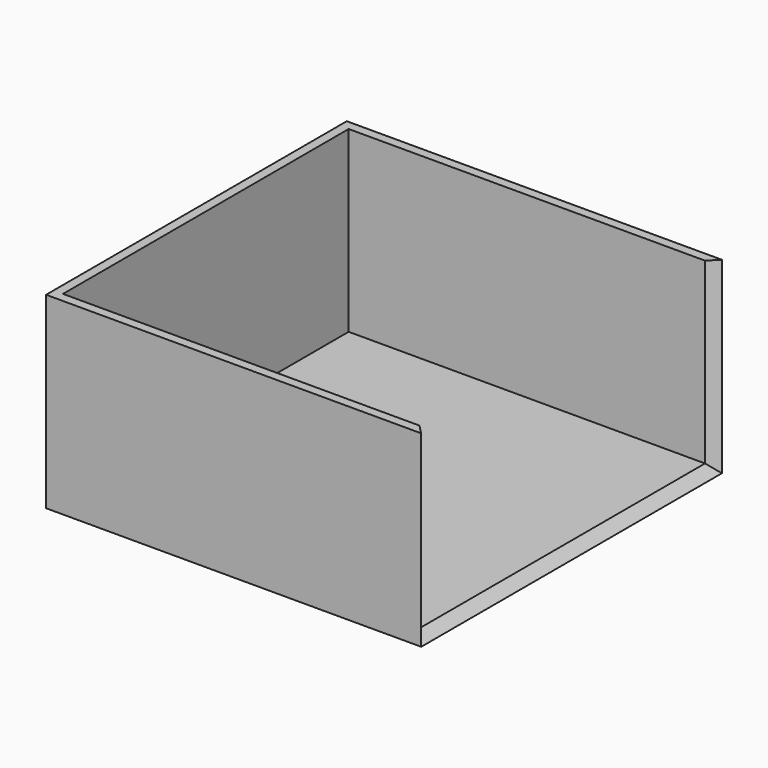
from build123d import *

# Parameters (mm, degrees)
F0_W         = 127
F0_H         = 127
F1_DEPTH     = 63.5
F2_W         = 120.65
F2_H         = 120.65
F2_W_2       = 40.16652188
F3_DEPTH     = 60.325
F4_T1_DEPTH  = 69.1433009657
F4_T3_DEPTH  = 120.65
F4_T9_DEPTH  = 129.4683009657
F4_T15_DEPTH = 69.1433009657
F4_T24_DEPTH = 69.1433009657
F4_T30_DEPTH = 129.4683009657


# Not quite as in the source:
# - a fillet or chamfer that OpenCascade refuses, or shapes differently, is made with other operations: its cross-section is extruded or revolved along the edge and cut away or added


with BuildPart() as f1:
    # F0 (on Top) → F1 (new body)
    with BuildSketch(Plane.XY):
        with Locations((9.8422262818, 3.4245376295)):
            Rectangle(F0_W, F0_H)
    extrude(amount=F1_DEPTH)

    # F2 (on face) → F3 (cut)
    with BuildSketch(Plane.XY.offset(63.5)):
        with Locations((9.8422262818, 3.4245376295)):
            Rectangle(F2_W, F2_H)
        with Locations((90.2504872218, 3.4245376295)):
            Rectangle(F2_W_2, F2_H)
    extrude(amount=-F3_DEPTH, mode=Mode.SUBTRACT)

    # F4: chamfer of 3.429 on 3 edges, made by hand

    # F4_s2 → F4_t1 (cut)
    with BuildSketch(Plane.XY.offset(3.175)):
        Polygon((73.3422262818, -60.3294623705), (69.9132262818, -56.9004623705), (73.3422262818, -56.9004623705), align=None)
        Polygon((73.3422262818, 67.1785376295), (69.9132262818, 63.7495376295), (73.3422262818, 63.7495376295), align=None)
    extrude(amount=F4_T1_DEPTH, mode=Mode.SUBTRACT)

    # F4_s4 → F4_t3 (cut)
    with BuildSketch(Plane.XZ.offset(-63.7495376295)):
        Polygon((73.3422262818, -0.254), (69.9132262818, 3.175), (73.3422262818, 3.175), align=None)
    extrude(amount=F4_T3_DEPTH, mode=Mode.SUBTRACT)


with BuildPart() as f4_tool7:
    # F4_s8 → F4_t9 (new body)
    with BuildSketch(Plane.XZ.offset(65.7187633362)):
        Polygon((73.3422262818, -0.254), (69.9132262818, 3.175), (73.3422262818, 3.175), align=None)
    extrude(amount=-F4_T9_DEPTH)

    split(bisect_by=Plane.XZ.offset(60.0754623705), keep=Keep.BOTTOM)

    split(bisect_by=Plane.XY, keep=Keep.TOP)

    split(bisect_by=Plane.XZ.offset(56.9004623705), keep=Keep.TOP)


with BuildPart() as f4_tool13:
    # F4_s14 → F4_t15 (new body)
    with BuildSketch(Plane.XY.offset(-5.6433009657)):
        Polygon((73.3422262818, -60.3294623705), (69.9132262818, -56.9004623705), (73.3422262818, -56.9004623705), align=None)
    extrude(amount=F4_T15_DEPTH)

    split(bisect_by=Plane.XZ.offset(60.0754623705), keep=Keep.BOTTOM)

    split(bisect_by=Plane.XY, keep=Keep.TOP)

    split(bisect_by=Plane.XY.offset(3.175), keep=Keep.BOTTOM)


with BuildPart() as f4_tool7_1:
    add(f4_tool7.part)

    # F4_t19: intersect F4_tool13
    add(f4_tool13.part, mode=Mode.INTERSECT)


with BuildPart() as f1_1:
    add(f1.part)

    # F4_t5: cut F4_tool7
    add(f4_tool7_1.part, mode=Mode.SUBTRACT)


with BuildPart() as f4_tool22:
    # F4_s23 → F4_t24 (new body)
    with BuildSketch(Plane.XY.offset(63.5)):
        Polygon((73.3422262818, 67.1785376295), (69.9132262818, 63.7495376295), (73.3422262818, 63.7495376295), align=None)
    extrude(amount=-F4_T24_DEPTH)

    split(bisect_by=Plane.XY, keep=Keep.TOP)

    split(bisect_by=Plane.XZ.offset(-66.9245376295), keep=Keep.TOP)

    split(bisect_by=Plane.XY.offset(3.175), keep=Keep.BOTTOM)


with BuildPart() as f4_tool28:
    # F4_s29 → F4_t30 (new body)
    with BuildSketch(Plane.XZ.offset(56.9004623705)):
        Polygon((73.3422262818, -0.254), (69.9132262818, 3.175), (73.3422262818, 3.175), align=None)
    extrude(amount=-F4_T30_DEPTH)

    split(bisect_by=Plane.XY, keep=Keep.TOP)

    split(bisect_by=Plane.XZ.offset(-66.9245376295), keep=Keep.TOP)

    split(bisect_by=Plane.XZ.offset(-63.7495376295), keep=Keep.BOTTOM)


with BuildPart() as f4_tool22_1:
    add(f4_tool22.part)

    # F4_t34: intersect F4_tool28
    add(f4_tool28.part, mode=Mode.INTERSECT)


with BuildPart() as f1_2:
    add(f1_1.part)

    # F4_t20: cut F4_tool22
    add(f4_tool22_1.part, mode=Mode.SUBTRACT)


solid = f1_2.part
